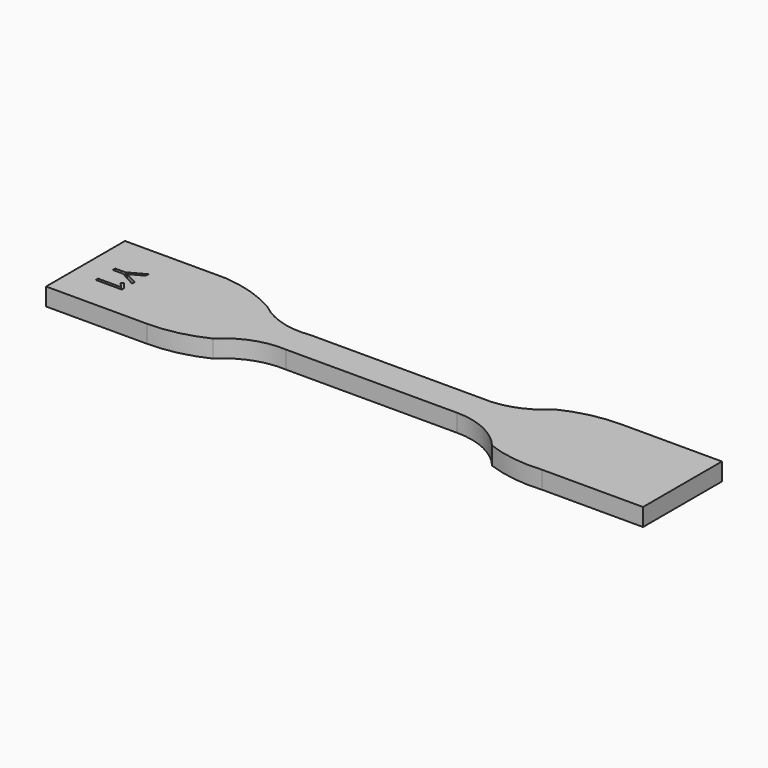
from build123d import *

# Parameters (mm, degrees)
F1_DEPTH     = 3.4
F2_TEXT_SIZE = 7.0564552314
F3_DEPTH     = 1


# Not quite as in the source:
# - Text() gives the source's letters only with a copy of the font that has no kerning and outlines rounded to 1/6400 em; it was checked with that copy


with BuildPart() as f1:
    # F0 (on Top) → F1 (new body)
    with BuildSketch(Plane.XY):
        with BuildLine():
            Line((-14.4320548165, 19.7811394548), (-33.8720548165, 19.7811394548))
            Line((-33.8720548165, 19.7811394548), (-33.8720548165, 0.7811394548))
            Line((-33.8720548165, 0.7811394548), (-14.4320548165, 0.7811394548))
            ThreePointArc((-14.4320548165, 0.7811394548), (-8.9053122052, 1.3996892086), (-3.6520548165, 3.2247301661))
            ThreePointArc((-3.6520548165, 3.2247301661), (1.3014698263, 6.4128780055), (7.1279451835, 7.2811394548))
            Line((7.1279451835, 7.2811394548), (40.1279451835, 7.2811394548))
            ThreePointArc((40.1279451835, 7.2811394548), (46.0837574042, 5.9511158081), (50.9079451835, 2.2137538538))
            ThreePointArc((50.9079451835, 2.2137538538), (56.2191047011, 0.9041953221), (61.6879451835, 0.7811394548))
            Line((61.6879451835, 0.7811394548), (81.1279451835, 0.7811394548))
            Line((81.1279451835, 0.7811394548), (81.1279451835, 19.7811394548))
            Line((81.1279451835, 19.7811394548), (61.6879451835, 19.7811394548))
            ThreePointArc((61.6879451835, 19.7811394548), (56.1612025723, 19.162589701), (50.9079451835, 17.3375487435))
            ThreePointArc((50.9079451835, 17.3375487435), (45.9544205407, 14.1494009041), (40.1279451835, 13.2811394548))
            Line((40.1279451835, 13.2811394548), (7.1279451835, 13.2811394548))
            ThreePointArc((7.1279451835, 13.2811394548), (1.4167452884, 13.6925537245), (-3.6520548165, 16.3560723447))
            ThreePointArc((-3.6520548165, 16.3560723447), (-8.8458057958, 18.686276846), (-14.4320548165, 19.7811394548))
        make_face()
    extrude(amount=F1_DEPTH)

    # F2 (on face) → F3 (cut)
    with BuildSketch(Plane.XY.offset(3.4)):
        with Locations(Location((-29.3886531144, 13.5272191837), (0, 0, -90))):
            Text('Y1', F2_TEXT_SIZE, font='Open Sans', text_align=(TextAlign.LEFT, TextAlign.BOTTOM))
    extrude(amount=-F3_DEPTH, mode=Mode.SUBTRACT)


solid = f1.part
